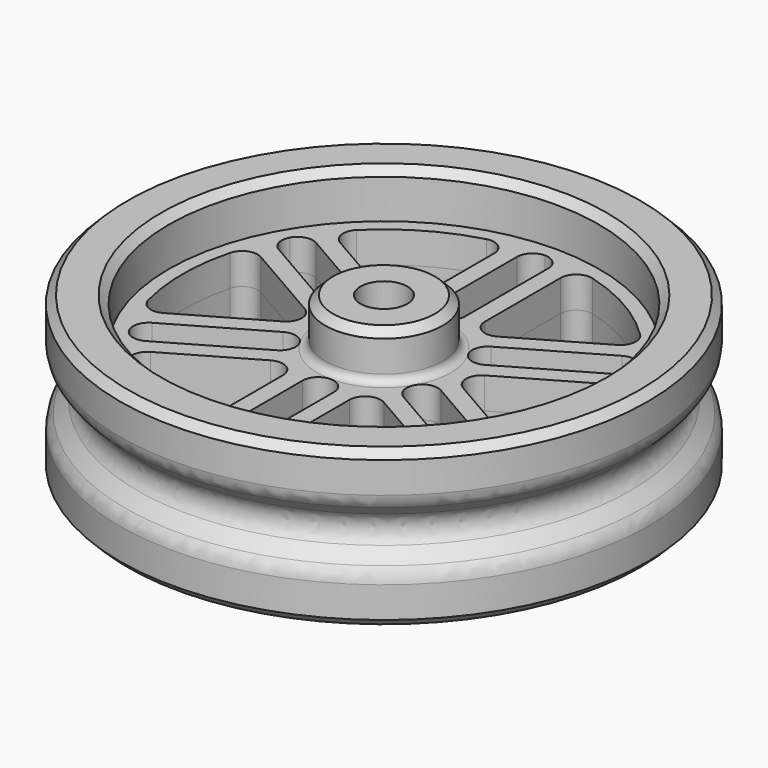
from build123d import *

# Parameters (mm, degrees)
F0_R     = 67.5
F0_R_2   = 55
F1_DEPTH = 12
F0_R_3   = 15
F2_DEPTH = 8
F0_R_4   = 6
F3_DEPTH = 12
F4_DEPTH = 8
F6_DEPTH = 8
F8_SIZE2 = 7.99999
F8_SIZE  = 7.99999
F10_R    = 5
F11_SIZE = 2
F12_R    = 4
F13_R    = 4
F14_R    = 1.99999


# Not quite as in the source:
# - a fillet or chamfer is up to 0.001 mm smaller than in the source, because OpenCascade refuses the exact size


with BuildPart() as f1:
    # F0 (on Top) → F1 (new body)
    with BuildSketch(Plane.XY):
        Circle(F0_R)
        Circle(F0_R_2, mode=Mode.SUBTRACT)
    extrude(amount=F1_DEPTH)

    # F0 (on Top) → F2 (join)
    with BuildSketch(Plane.XY):
        Circle(F0_R_2)
        with BuildLine():
            ThreePointArc((48.2386348958, 18.0356342662), (50.6781002857, 9.1640684978), (51.5, 0))
            ThreePointArc((51.5, 0), (50.6781002857, -9.1640684978), (48.2386348958, -18.0356342662))
            ThreePointArc((48.2386348958, -18.0356342662), (46.5794503909, -21.9682680538), (44.6003081906, -25.7500001806))
            ThreePointArc((44.6003081906, -25.7500001806), (42.3148032883, -29.3548534773), (39.7386348958, -32.7580661306))
            ThreePointArc((39.7386348958, -32.7580661306), (25.75, -44.6003082949), (8.5, -50.7937003968))
            ThreePointArc((8.5, -50.7937003968), (4.2646470273, -51.3231213561), (-1.211e-07, -51.5))
            ThreePointArc((-1.211e-07, -51.5), (-4.264647148, -51.3231213461), (-8.5, -50.7937003968))
            ThreePointArc((-8.5, -50.7937003968), (-25.75, -44.6003082949), (-39.7386348958, -32.7580661306))
            ThreePointArc((-39.7386348958, -32.7580661306), (-42.3148034084, -29.3548533041), (-44.6003084014, -25.7499998155))
            ThreePointArc((-44.6003084014, -25.7499998155), (-46.5794504808, -21.9682678631), (-48.2386348958, -18.0356342662))
            ThreePointArc((-48.2386348958, -18.0356342662), (-51.5, 0), (-48.2386348958, 18.0356342662))
            ThreePointArc((-48.2386348958, 18.0356342662), (-46.5794504341, 21.9682679622), (-44.6003082919, 25.7500000053))
            ThreePointArc((-44.6003082919, 25.7500000053), (-42.314803346, 29.3548533941), (-39.7386348958, 32.7580661306))
            ThreePointArc((-39.7386348958, 32.7580661306), (-25.75, 44.6003082949), (-8.5, 50.7937003968))
            ThreePointArc((-8.5, 50.7937003968), (-4.2646470845, 51.3231213513), (6.3e-09, 51.5))
            ThreePointArc((6.3e-09, 51.5), (4.2646470908, 51.3231213508), (8.5, 50.7937003968))
            ThreePointArc((8.5, 50.7937003968), (25.75, 44.6003082949), (39.7386348958, 32.7580661306))
            ThreePointArc((39.7386348958, 32.7580661306), (42.314803346, 29.3548533941), (44.6003082919, 25.7500000053))
            ThreePointArc((44.6003082919, 25.7500000053), (46.5794504341, 21.9682679622), (48.2386348958, 18.0356342662))
        make_face(mode=Mode.SUBTRACT)
        with BuildLine():
            Line((17, 0), (48.2386348958, 18.0356342662))
            ThreePointArc((48.2386348958, 18.0356342662), (46.5794504341, 21.9682679622), (44.6003082919, 25.7500000053))
            ThreePointArc((44.6003082919, 25.7500000053), (42.314803346, 29.3548533941), (39.7386348958, 32.7580661306))
            Line((39.7386348958, 32.7580661306), (8.5, 14.7224318643))
            Line((8.5, 14.7224318643), (8.5, 50.7937003968))
            ThreePointArc((8.5, 50.7937003968), (4.2646470908, 51.3231213508), (6.3e-09, 51.5))
            ThreePointArc((6.3e-09, 51.5), (-4.2646470845, 51.3231213513), (-8.5, 50.7937003968))
            Line((-8.5, 50.7937003968), (-8.5, 14.7224318643))
            Line((-8.5, 14.7224318643), (-39.7386348958, 32.7580661306))
            ThreePointArc((-39.7386348958, 32.7580661306), (-42.314803346, 29.3548533941), (-44.6003082919, 25.7500000053))
            ThreePointArc((-44.6003082919, 25.7500000053), (-46.5794504341, 21.9682679622), (-48.2386348958, 18.0356342662))
            Line((-48.2386348958, 18.0356342662), (-17, 0))
            Line((-17, 0), (-48.2386348958, -18.0356342662))
            ThreePointArc((-48.2386348958, -18.0356342662), (-46.5794504808, -21.9682678631), (-44.6003084014, -25.7499998155))
            ThreePointArc((-44.6003084014, -25.7499998155), (-42.3148034084, -29.3548533041), (-39.7386348958, -32.7580661306))
            Line((-39.7386348958, -32.7580661306), (-8.5, -14.7224318643))
            Line((-8.5, -14.7224318643), (-8.5, -50.7937003968))
            ThreePointArc((-8.5, -50.7937003968), (-4.264647148, -51.3231213461), (-1.211e-07, -51.5))
            ThreePointArc((-1.211e-07, -51.5), (4.2646470273, -51.3231213561), (8.5, -50.7937003968))
            Line((8.5, -50.7937003968), (8.5, -14.7224318643))
            Line((8.5, -14.7224318643), (39.7386348958, -32.7580661306))
            ThreePointArc((39.7386348958, -32.7580661306), (42.3148032883, -29.3548534773), (44.6003081906, -25.7500001806))
            ThreePointArc((44.6003081906, -25.7500001806), (46.5794503909, -21.9682680538), (48.2386348958, -18.0356342662))
            Line((48.2386348958, -18.0356342662), (17, 0))
        make_face()
        with BuildLine():
            ThreePointArc((-39.1362066798, -27.2141016151), (-42.171482963, -27.6137032776), (-44.6003084014, -25.7499998155))
            ThreePointArc((-44.6003084014, -25.7499998155), (-44.9999099574, -22.7147237167), (-43.1362066798, -20.2858983849))
            Line((-43.1362066798, -20.2858983849), (-20.1865334795, -7.0358983849))
            ThreePointArc((-20.1865334795, -7.0358983849), (-16.1865334795, -7.0358983849), (-14.1865334795, -10.5))
            ThreePointArc((-14.1865334795, -10.5), (-14.7224318643, -12.5), (-16.1865334795, -13.9641016151))
            Line((-16.1865334795, -13.9641016151), (-39.1362066798, -27.2141016151))
        make_face(mode=Mode.SUBTRACT)
        with BuildLine():
            ThreePointArc((4, -47.5), (2.8284270819, -50.3284271676), (-1.211e-07, -51.5))
            ThreePointArc((-1.211e-07, -51.5), (-2.8284271676, -50.3284270819), (-4, -47.5))
            Line((-4, -47.5), (-4, -21))
            ThreePointArc((-4, -21), (0, -17), (4, -21))
            Line((4, -21), (4, -47.5))
        make_face(mode=Mode.SUBTRACT)
        with BuildLine():
            ThreePointArc((45.1362066798, -23.75), (44.9999099579, -24.7852762812), (44.6003081906, -25.7500001806))
            ThreePointArc((44.6003081906, -25.7500001806), (42.1714827594, -27.6137033322), (39.1362066798, -27.2141016151))
            Line((39.1362066798, -27.2141016151), (16.1865334795, -13.9641016151))
            ThreePointArc((16.1865334795, -13.9641016151), (14.7224318643, -8.5), (20.1865334795, -7.0358983849))
            Line((20.1865334795, -7.0358983849), (43.1362066798, -20.2858983849))
            ThreePointArc((43.1362066798, -20.2858983849), (44.6003082949, -21.75), (45.1362066798, -23.75))
        make_face(mode=Mode.SUBTRACT)
        with BuildLine():
            ThreePointArc((-43.1362066798, 20.2858983849), (-44.9999099857, 22.7147238225), (-44.6003082919, 25.7500000053))
            ThreePointArc((-44.6003082919, 25.7500000053), (-42.1714828572, 27.6137033059), (-39.1362066798, 27.2141016151))
            Line((-39.1362066798, 27.2141016151), (-16.1865334795, 13.9641016151))
            ThreePointArc((-16.1865334795, 13.9641016151), (-14.7224318643, 12.5), (-14.1865334795, 10.5))
            ThreePointArc((-14.1865334795, 10.5), (-16.1865334795, 7.0358983849), (-20.1865334795, 7.0358983849))
            Line((-20.1865334795, 7.0358983849), (-43.1362066798, 20.2858983849))
        make_face(mode=Mode.SUBTRACT)
        Circle(F0_R_3, mode=Mode.SUBTRACT)
        with BuildLine():
            ThreePointArc((39.1362066798, 27.2141016151), (42.1714828572, 27.6137033059), (44.6003082919, 25.7500000053))
            ThreePointArc((44.6003082919, 25.7500000053), (44.9999099841, 24.7852761833), (45.1362066798, 23.75))
            ThreePointArc((45.1362066798, 23.75), (44.6003082949, 21.75), (43.1362066798, 20.2858983849))
            Line((43.1362066798, 20.2858983849), (20.1865334795, 7.0358983849))
            ThreePointArc((20.1865334795, 7.0358983849), (14.7224318643, 8.5), (16.1865334795, 13.9641016151))
            Line((16.1865334795, 13.9641016151), (39.1362066798, 27.2141016151))
        make_face(mode=Mode.SUBTRACT)
        with BuildLine():
            ThreePointArc((-4, 47.5), (-2.8284271225, 50.328427127), (6.3e-09, 51.5))
            ThreePointArc((6.3e-09, 51.5), (2.828427127, 50.3284271225), (4, 47.5))
            Line((4, 47.5), (4, 21))
            ThreePointArc((4, 21), (0, 17), (-4, 21))
            Line((-4, 21), (-4, 47.5))
        make_face(mode=Mode.SUBTRACT)
    extrude(amount=-F2_DEPTH)

    # F0 (on Top) → F3 (join)
    with BuildSketch(Plane.XY):
        Circle(F0_R_3)
        Circle(F0_R_4, mode=Mode.SUBTRACT)
    extrude(amount=F3_DEPTH)

    # F0 (on Top) → F4 (join)
    with BuildSketch(Plane.XY):
        Circle(F0_R_3)
        Circle(F0_R_4, mode=Mode.SUBTRACT)
    extrude(amount=-F4_DEPTH)

    # F5: union 

    # F0 (on Top) → F6 (join)
    with BuildSketch(Plane.XY):
        Circle(F0_R)
        Circle(F0_R_2, mode=Mode.SUBTRACT)
    extrude(amount=-F6_DEPTH)

    # F7: union 

    # F8 (size 8 and 8 in the source; OpenCascade refuses exactly that, so slightly less here)
    f8_edges = [f1.edges().sort_by_distance(p)[0] for p in [
        (-67.5, 0, -8),
    ]]
    chamfer(f8_edges, length=F8_SIZE, length2=F8_SIZE2)

    # F9: F1 across face


with BuildPart() as f1_1:
    add(f1.part)
    add(f1.part.mirror(Plane(origin=(0, 0, -8), x_dir=(1, 0, 0), z_dir=(0, 0, -1))))

    # F10
    f10_edges = [f1_1.edges().sort_by_distance(p)[0] for p in [
        (-59.50001, 0, -8),
        (-67.5, 0, -16),
        (-67.5, 0, -15.99999),
        (-67.5, 0, -1e-05),
    ]]
    fillet(f10_edges, radius=F10_R)

    # F11
    f11_edges = [f1_1.edges().sort_by_distance(p)[0] for p in [
        (-67.5, 0, 12),
        (-67.5, 0, -28),
        (-55, 0, -28),
        (-15, 0, -28),
        (-55, 0, 12),
        (-15, 0, 12),
    ]]
    chamfer(f11_edges, length=F11_SIZE)

    # F12
    f12_edges = [f1_1.edges().sort_by_distance(p)[0] for p in [
        (-39.738635, 32.758066, -4),
        (-39.738635, 32.758066, -12),
        (-48.238635, 18.035634, -4),
        (-48.238635, 18.035634, -12),
        (8.5, 50.7937, -4),
        (8.5, 50.7937, -12),
        (48.238635, 18.035634, -4),
        (48.238635, 18.035634, -12),
        (39.738635, 32.758066, -4),
        (39.738635, 32.758066, -12),
        (39.738635, -32.758066, -4),
        (39.738635, -32.758066, -12),
        (48.238635, -18.035634, -4),
        (48.238635, -18.035634, -12),
        (-8.5, -50.7937, -4),
        (-8.5, -50.7937, -12),
        (8.5, -50.7937, -4),
        (8.5, -50.7937, -12),
        (-48.238635, -18.035634, -4),
        (-48.238635, -18.035634, -12),
        (-39.738635, -32.758066, -4),
        (-39.738635, -32.758066, -12),
        (-8.5, 50.7937, -4),
        (-8.5, 50.7937, -12),
    ]]
    fillet(f12_edges, radius=F12_R)

    # F13
    f13_edges = [f1_1.edges().sort_by_distance(p)[0] for p in [
        (8.5, -14.722432, -4),
        (8.5, -14.722432, -12),
        (17, 0, -4),
        (17, 0, -12),
        (8.5, 14.722432, -4),
        (8.5, 14.722432, -12),
        (-8.5, 14.722432, -4),
        (-8.5, 14.722432, -12),
        (-17, 0, -4),
        (-17, 0, -12),
        (-8.5, -14.722432, -4),
        (-8.5, -14.722432, -12),
    ]]
    fillet(f13_edges, radius=F13_R)

    # F14 (radius 2 in the source; OpenCascade refuses exactly that, so slightly less here)
    f14_edges = [f1_1.edges().sort_by_distance(p)[0] for p in [
        (-15, 0, 0),
        (-15, 0, -16),
    ]]
    fillet(f14_edges, radius=F14_R)


solid = f1_1.part
